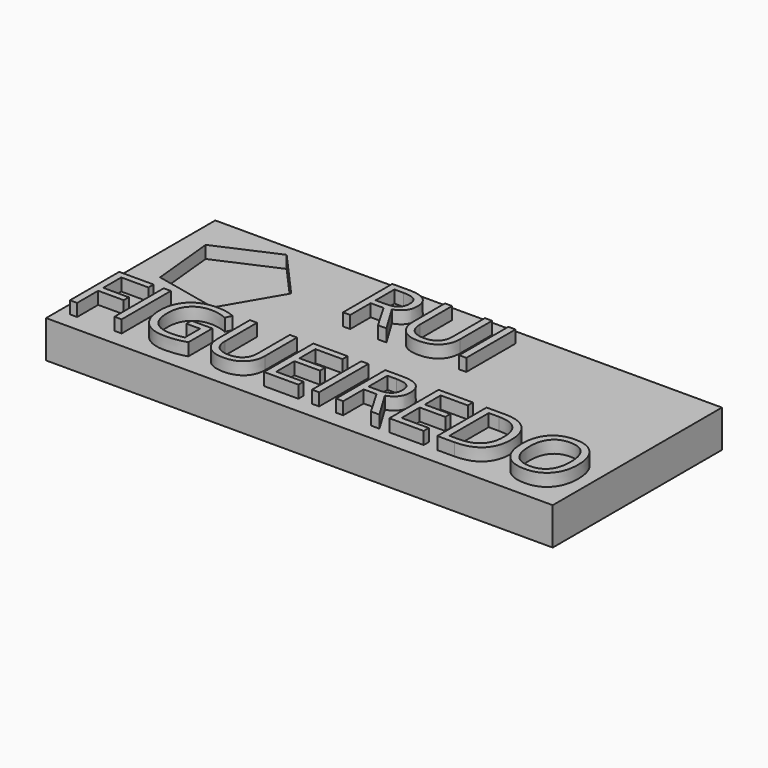
from build123d import *

# Parameters (mm, degrees)
F0_W         = 101.7987802625
F0_H         = 42.4961913377
F1_DEPTH     = 7.5
F4_DEPTH     = 2.5
F2_TEXT_SIZE = 17.326330608
F5_DEPTH     = 2.5


# Not quite as in the source:
# - Text() gives the source's letters only with a copy of the font that has no kerning and outlines rounded to 1/6400 em; it was checked with that copy


with BuildPart() as f1:
    # F0 (on Top) → F1 (new body)
    with BuildSketch(Plane.XY):
        with Locations((1.7682462931, 0.0326774316)):
            Rectangle(F0_W, F0_H)
    extrude(amount=F1_DEPTH)

    # F3 (on face) → F4 (cut)
    with BuildSketch(Plane.XY.offset(7.5)):
        Polygon((-30.9523434056, -2.0323234688), (-24.3225199359, 9.3289566512), (-33.0790113057, 19.1451220988), (-45.120644064, 13.8505658647), (-43.806291019, 0.762184709), align=None)
    extrude(amount=-F4_DEPTH, mode=Mode.SUBTRACT)

    # F2 (on face) → F5 (join)
    with BuildSketch(Plane.XY.offset(7.5)):
        with Locations((-12.6638495809, 5.661366362)):
            Text('RUI', F2_TEXT_SIZE, font='Open Sans', text_align=(TextAlign.LEFT, TextAlign.BOTTOM))
        with Locations((-48.6809593323, -17.9024432649)):
            Text('FIGUEIREDO', F2_TEXT_SIZE, font='Open Sans', text_align=(TextAlign.LEFT, TextAlign.BOTTOM))
    extrude(amount=F5_DEPTH)


solid = f1.part
